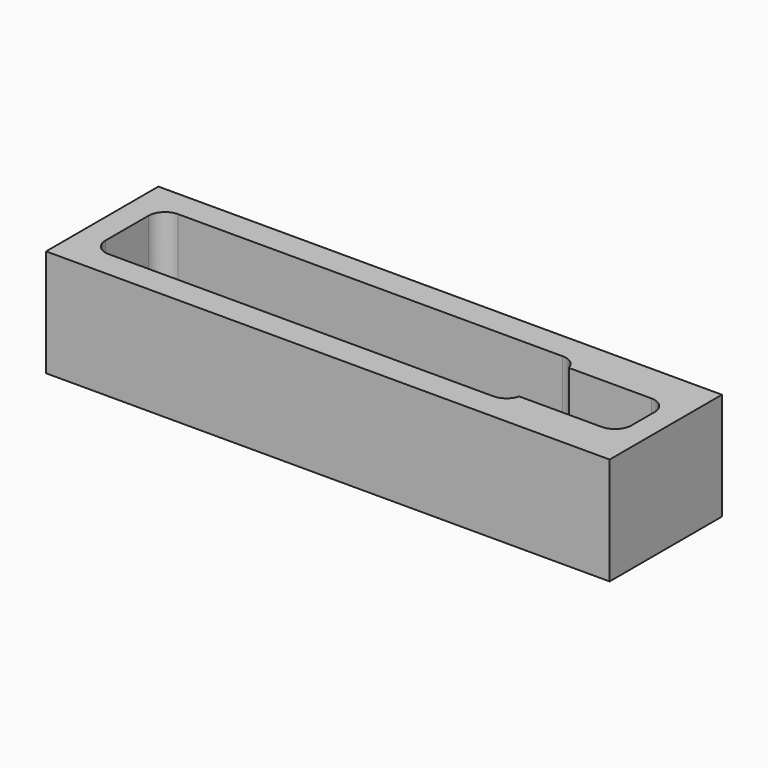
from build123d import *

# Parameters (mm, degrees)
F0_W         = 254
F0_H         = 53.975
F1_DEPTH     = 41.275
F3_DEPTH     = 22.225
F4_T1_DEPTH  = 38.1
F4_T3_DEPTH  = 37.5959026553
F6_DEPTH     = 11.43
F8_DEPTH     = 41.276
F9_T1_DEPTH  = 19.05
F9_T3_DEPTH  = 7.62
F10_W        = 37.30625
F10_H        = 41.275
F11_DEPTH    = 53.976
F12_W        = 19.05
F12_H        = 2.38125
F13_DEPTH    = 3.175
F14_T1_DEPTH = 15.5674179031


# Not quite as in the source:
# - a fillet or chamfer that OpenCascade refuses, or shapes differently, is made with other operations: its cross-section is extruded or revolved along the edge and cut away or added


with BuildPart() as f1:
    # F0 (on Top) → F1 (new body)
    with BuildSketch(Plane.XY):
        Rectangle(F0_W, F0_H)
    extrude(amount=F1_DEPTH)

    # F2 (on face) → F3 (cut)
    with BuildSketch(Plane.XY.offset(41.275)):
        Polygon((-80.16875, 16.66875), (-80.16875, -16.66875), (80.16875, -16.66875), (80.16875, -11.90625), (118.26875, -11.90625), (118.26875, 11.90625), (80.16875, 11.90625), (80.16875, 16.66875), align=None)
    extrude(amount=-F3_DEPTH, mode=Mode.SUBTRACT)

    # F4: fillet of radius 6.35 on 6 edges, made by hand

    # F4_s2 → F4_t1 (join)
    with BuildSketch(Plane.XY.offset(3.175)):
        with BuildLine():
            ThreePointArc((-80.16875, -10.31875), (-78.3088780605, -14.8088780605), (-73.81875, -16.66875))
            Line((-73.81875, -16.66875), (-80.16875, -16.66875))
            Line((-80.16875, -16.66875), (-80.16875, -10.31875))
        make_face()
        with BuildLine():
            ThreePointArc((111.91875, -11.90625), (116.4088780605, -10.0463780605), (118.26875, -5.55625))
            Line((118.26875, -5.55625), (118.26875, -11.90625))
            Line((118.26875, -11.90625), (111.91875, -11.90625))
        make_face()
        with BuildLine():
            ThreePointArc((118.26875, 5.55625), (116.4088780605, 10.0463780605), (111.91875, 11.90625))
            Line((111.91875, 11.90625), (118.26875, 11.90625))
            Line((118.26875, 11.90625), (118.26875, 5.55625))
        make_face()
        with BuildLine():
            ThreePointArc((-80.16875, 10.31875), (-78.3088780605, 14.8088780605), (-73.81875, 16.66875))
            Line((-73.81875, 16.66875), (-80.16875, 16.66875))
            Line((-80.16875, 16.66875), (-80.16875, 10.31875))
        make_face()
    extrude(amount=F4_T1_DEPTH)

    # F4_s4 → F4_t3 (join)
    with BuildSketch(Plane.XY.offset(3.6790973447)):
        with BuildLine():
            ThreePointArc((80.16875, 11.90625), (77.9089539046, 15.3388657855), (74.0203889379, 16.66875))
            Line((74.0203889379, 16.66875), (80.16875, 16.66875))
            Line((80.16875, 16.66875), (80.16875, 11.90625))
        make_face()
        with BuildLine():
            ThreePointArc((74.0203889379, -16.66875), (77.9089539046, -15.3388657855), (80.16875, -11.90625))
            Line((80.16875, -11.90625), (80.16875, -16.66875))
            Line((80.16875, -16.66875), (74.0203889379, -16.66875))
        make_face()
    extrude(amount=F4_T3_DEPTH)

    # F5 (on face) → F6 (cut)
    with BuildSketch(Plane(origin=(0, 0, 0), x_dir=(1, 0, 0), z_dir=(0, 0, -1))):
        with BuildLine():
            Line((-29.36875, 9.525), (-70.64375, 9.525))
            ThreePointArc((-70.64375, 9.525), (-80.16875, 0), (-70.64375, -9.525))
            Line((-70.64375, -9.525), (-29.36875, -9.525))
            Line((-29.36875, -9.525), (-29.36875, -11.90625))
            Line((-29.36875, -11.90625), (3.96875, -11.90625))
            Line((3.96875, -11.90625), (3.96875, -16.66875))
            Line((3.96875, -16.66875), (67.3851976236, -16.66875))
            Line((67.3851976236, -16.66875), (67.3851976236, 16.66875))
            Line((67.3851976236, 16.66875), (3.96875, 16.66875))
            Line((3.96875, 16.66875), (3.96875, 11.90625))
            Line((3.96875, 11.90625), (-29.36875, 11.90625))
            Line((-29.36875, 11.90625), (-29.36875, 9.525))
        make_face()
    extrude(amount=-F6_DEPTH, mode=Mode.SUBTRACT)

    # F7 (on face) → F8 (cut, through all)
    with BuildSketch(Plane(origin=(0, 0, 0), x_dir=(1, 0, 0), z_dir=(0, 0, -1))):
        with BuildLine():
            Line((-29.36875, 9.525), (-70.64375, 9.525))
            ThreePointArc((-70.64375, 9.525), (-72.2544463474, 9.3878262807), (-73.81875, 8.9802561211))
            Line((-73.81875, 8.9802561211), (-73.81875, -8.9802561211))
            ThreePointArc((-73.81875, -8.9802561211), (-72.2544463474, -9.3878262807), (-70.64375, -9.525))
            Line((-70.64375, -9.525), (-29.36875, -9.525))
            Line((-29.36875, -9.525), (-29.36875, -11.90625))
            Line((-29.36875, -11.90625), (3.96875, -11.90625))
            Line((3.96875, -11.90625), (3.96875, -16.66875))
            Line((3.96875, -16.66875), (67.3851976236, -16.66875))
            Line((67.3851976236, -16.66875), (67.3851976236, 16.66875))
            Line((67.3851976236, 16.66875), (3.96875, 16.66875))
            Line((3.96875, 16.66875), (3.96875, 11.90625))
            Line((3.96875, 11.90625), (-29.36875, 11.90625))
            Line((-29.36875, 11.90625), (-29.36875, 9.525))
        make_face()
    extrude(amount=-F8_DEPTH, mode=Mode.SUBTRACT)

    # F9: fillet of radius 6.35 on 8 edges, made by hand

    # F9_s2 → F9_t1 (join)
    with BuildSketch(Plane.XY):
        with BuildLine():
            ThreePointArc((3.96875, -11.90625), (6.2285460954, -15.3388657855), (10.1171110621, -16.66875))
            Line((10.1171110621, -16.66875), (3.96875, -16.66875))
            Line((3.96875, -16.66875), (3.96875, -11.90625))
        make_face()
        with BuildLine():
            ThreePointArc((-24.4117828388, -11.90625), (-27.1614134958, -11.2800626498), (-29.36875, -9.525))
            Line((-29.36875, -9.525), (-29.36875, -11.90625))
            Line((-29.36875, -11.90625), (-24.4117828388, -11.90625))
        make_face()
        with BuildLine():
            ThreePointArc((61.0351976236, -16.66875), (65.5253256842, -14.8088780605), (67.3851976236, -10.31875))
            Line((67.3851976236, -10.31875), (67.3851976236, -16.66875))
            Line((67.3851976236, -16.66875), (61.0351976236, -16.66875))
        make_face()
        with BuildLine():
            ThreePointArc((67.3851976236, 10.31875), (65.5253256842, 14.8088780605), (61.0351976236, 16.66875))
            Line((61.0351976236, 16.66875), (67.3851976236, 16.66875))
            Line((67.3851976236, 16.66875), (67.3851976236, 10.31875))
        make_face()
        with BuildLine():
            ThreePointArc((3.96875, 11.90625), (6.2285460954, 15.3388657855), (10.1171110621, 16.66875))
            Line((10.1171110621, 16.66875), (3.96875, 16.66875))
            Line((3.96875, 16.66875), (3.96875, 11.90625))
        make_face()
        with BuildLine():
            ThreePointArc((-29.36875, 9.525), (-27.1614134958, 11.2800626498), (-24.4117828388, 11.90625))
            Line((-24.4117828388, 11.90625), (-29.36875, 11.90625))
            Line((-29.36875, 11.90625), (-29.36875, 9.525))
        make_face()
    extrude(amount=F9_T1_DEPTH)

    # F9_s4 → F9_t3 (join)
    with BuildSketch(Plane.XY.offset(11.43)):
        with BuildLine():
            ThreePointArc((-73.81875, 3.175), (-71.9588780605, 7.6651280605), (-67.46875, 9.525))
            Line((-67.46875, 9.525), (-67.46875, 10.16))
            ThreePointArc((-67.46875, 10.16), (-70.64375, 10.16), (-74.0304166667, 9.5789398625))
            Line((-74.0304166667, 9.5789398625), (-74.45375, 8.9802561211))
            Line((-74.45375, 8.9802561211), (-74.45375, 3.175))
            Line((-74.45375, 3.175), (-73.81875, 3.175))
        make_face()
        with BuildLine():
            ThreePointArc((-73.81875, -3.175), (-71.9588780605, -7.6651280605), (-67.46875, -9.525))
            Line((-67.46875, -9.525), (-67.46875, -10.16))
            ThreePointArc((-67.46875, -10.16), (-70.64375, -10.16), (-74.0304166667, -9.5789398625))
            Line((-74.0304166667, -9.5789398625), (-74.45375, -8.9802561211))
            Line((-74.45375, -8.9802561211), (-74.45375, -3.175))
            Line((-74.45375, -3.175), (-73.81875, -3.175))
        make_face()
    extrude(amount=F9_T3_DEPTH)

    # F10 (on face) → F11 (cut, through all)
    with BuildSketch(Plane.XZ.offset(26.9875)):
        with Locations((-108.346875, 20.6375)):
            Rectangle(F10_W, F10_H)
    extrude(amount=-F11_DEPTH, mode=Mode.SUBTRACT)

    # F12 (on face) → F13 (cut)
    with BuildSketch(Plane.XY.offset(19.05)):
        with Locations((-31.75, 10.715625)):
            Rectangle(F12_W, F12_H)
        with Locations((-31.75, -10.715625)):
            Rectangle(F12_W, F12_H)
    extrude(amount=-F13_DEPTH, mode=Mode.SUBTRACT)

    # F14: fillet of radius 6.35 on 2 edges, made by hand

    # F14_s2 → F14_t1 (join)
    with BuildSketch(Plane.XY.offset(3.4825820969)):
        with BuildLine():
            ThreePointArc((-41.275, 9.525), (-39.0676634958, 11.2800626498), (-36.3180328388, 11.90625))
            Line((-36.3180328388, 11.90625), (-41.275, 11.90625))
            Line((-41.275, 11.90625), (-41.275, 9.525))
        make_face()
        with BuildLine():
            ThreePointArc((-36.3180328388, -11.90625), (-39.0676634958, -11.2800626498), (-41.275, -9.525))
            Line((-41.275, -9.525), (-41.275, -11.90625))
            Line((-41.275, -11.90625), (-36.3180328388, -11.90625))
        make_face()
    extrude(amount=F14_T1_DEPTH)


solid = f1.part
